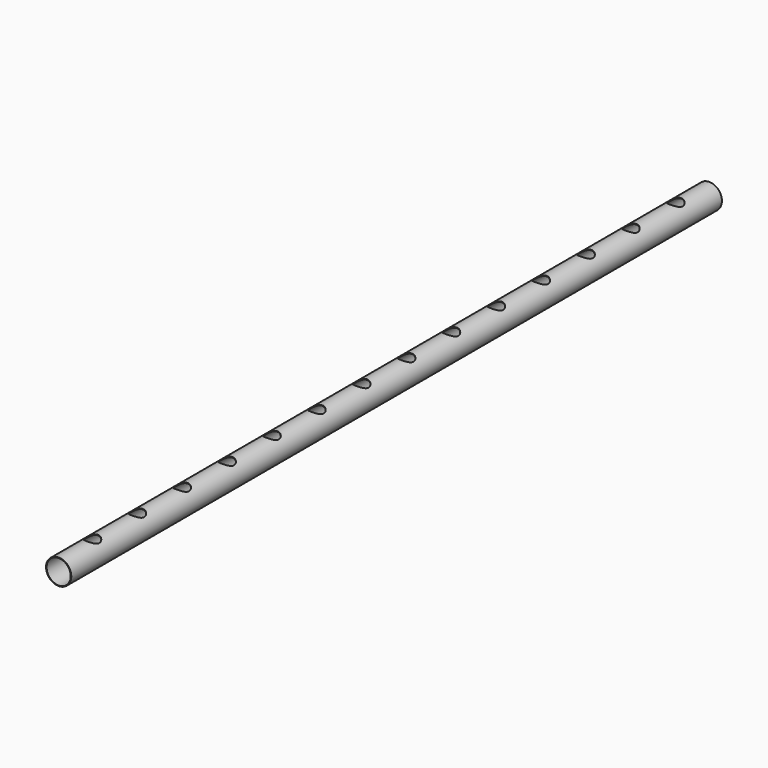
from build123d import *

# Parameters (mm, degrees)
F0_R     = 45
F0_R_2   = 43
F1_DEPTH = 1450
F4_D     = 50
F4_DEPTH = 50
F4_TIP   = 15.0215154757
F6_D     = 0.5
F6_DEPTH = 50
F6_TIP   = 0.1502151548


# Not quite as in the source:
# - a feature names something its author has since deleted; it is built from what else it names


with BuildPart() as f1:
    # F0 (on Front) → F1 (new body, symmetric)
    with BuildSketch(Plane.XZ):
        Circle(F0_R)
        Circle(F0_R_2, mode=Mode.SUBTRACT)
    extrude(amount=F1_DEPTH, both=True)

    # F4
    with Locations(Plane.XY.offset(45)):
        with Locations((0, -1300), (0, -1100), (0, -900), (0, -700), (0, -500), (0, -300), (0, -100), (0, 100), (0, 300), (0, 500), (0, 700), (0, 900), (0, 1100), (0, 1300)):
            Hole(F4_D / 2, depth=F4_DEPTH)
            with Locations((0, 0, -(F4_DEPTH + F4_TIP / 2))):  # 118° drill point
                Cone(0, F4_D / 2, F4_TIP, mode=Mode.SUBTRACT)

    # F6 (one way)
    with BuildSketch(Plane.XY):
        with Locations((0, 0)):
            Circle(F6_D / 2)
    extrude(amount=-F6_DEPTH, mode=Mode.SUBTRACT)
    with Locations(Plane.XY):
        with Locations((0, 0)):
            with Locations((0, 0, -(F6_DEPTH + F6_TIP / 2))):  # 118° drill point
                Cone(0, F6_D / 2, F6_TIP, mode=Mode.SUBTRACT)


solid = f1.part
